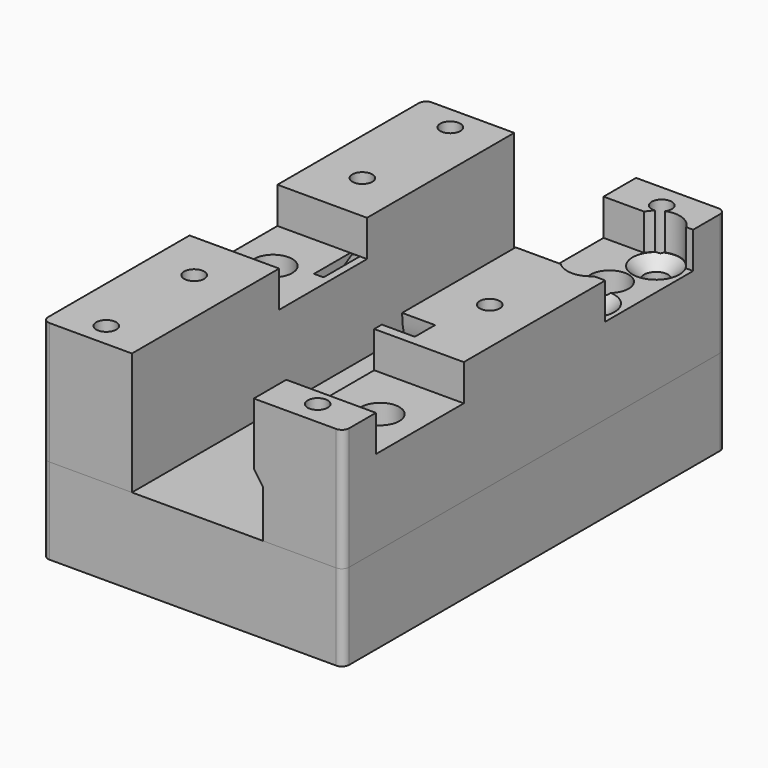
from build123d import *

# Parameters (mm, degrees)
F0_W      = 63
F0_H      = 100
F0_R      = 4
F1_DEPTH  = 25.6
F2_W      = 23
F2_H      = 7.6
F3_DEPTH  = 31.501
F4_W      = 23
F4_H      = 7.6
F5_DEPTH  = 31.501
F6_W      = 25.5
F6_H      = 100
F7_DEPTH  = 25.601
F8_R      = 4
F9_DEPTH  = 17
F10_R     = 2.1
F11_DEPTH = 29
F13_DEPTH = 100.001
F15_DEPTH = 15
F16_DEPTH = 5
F17_R     = 2.5
F18_DEPTH = 15.601
F20_DEPTH = 7.6
F22_R     = 1.5
F23_W     = 2
F23_H     = 20
F24_DEPTH = 18
F26_DEPTH = 6.5
F27_W     = 2
F27_H     = 20
F28_DEPTH = 3
F29_R     = 2.75
F30_DEPTH = 18
F31_R     = 3.4
F32_DEPTH = 43.6010001


# Not quite as in the source:
# - a fillet or chamfer that OpenCascade refuses, or shapes differently, is made with other operations: its cross-section is extruded or revolved along the edge and cut away or added


with BuildPart() as f1:
    # F0 (on Top) → F1 (new body)
    with BuildSketch(Plane.XY):
        Rectangle(F0_W, F0_H)
        with Locations((23.2, -30)):
            Circle(F0_R, mode=Mode.SUBTRACT)
        with Locations((-23.2, 0)):
            Circle(F0_R, mode=Mode.SUBTRACT)
        with Locations((23.2, 30)):
            Circle(F0_R, mode=Mode.SUBTRACT)
    extrude(amount=F1_DEPTH)

    # F2 (on Right) → F3 (cut, through all)
    with BuildSketch(Plane.YZ):
        with Locations((0, 21.8)):
            Rectangle(F2_W, F2_H)
    extrude(amount=-F3_DEPTH, mode=Mode.SUBTRACT)

    # F4 (on Right) → F5 (cut, through all)
    with BuildSketch(Plane.YZ):
        with Locations((-30, 21.8)):
            Rectangle(F4_W, F4_H)
        with Locations((30, 21.8)):
            Rectangle(F4_W, F4_H)
    extrude(amount=F5_DEPTH, mode=Mode.SUBTRACT)

    # F6 (on face) → F7 (cut, through all)
    with BuildSketch(Plane(origin=(0, 0, 0), x_dir=(1, 0, 0), z_dir=(0, 0, -1))):
        Rectangle(F6_W, F6_H)
    extrude(amount=-F7_DEPTH, mode=Mode.SUBTRACT)

    # F8 (on face) → F9 (cut)
    with BuildSketch(Plane(origin=(-31.5, 0, 0), x_dir=(0, -1, 0), z_dir=(-1, 0, 0))):
        with Locations((-12, 10)):
            Circle(F8_R)
    extrude(amount=-F9_DEPTH, mode=Mode.SUBTRACT)

    # F10 (on face) → F11 (cut)
    with BuildSketch(Plane.XY.offset(25.6)):
        with Locations((22.125, -45)):
            Circle(F10_R)
        with Locations((-22.125, -45)):
            Circle(F10_R)
        with Locations((22.125, 0)):
            Circle(F10_R)
        with Locations((-22.125, -22)):
            Circle(F10_R)
        with Locations((-22.125, 22)):
            Circle(F10_R)
        with Locations((-22.125, 45)):
            Circle(F10_R)
        with Locations((22.125, 45)):
            Circle(F10_R)
    extrude(amount=-F11_DEPTH, mode=Mode.SUBTRACT)

    # F12 (on face) → F13 (cut, through all)
    with BuildSketch(Plane.XZ.offset(50)):
        Polygon((12.75, 12.7134812128), (12.75, 0), (14.65, 0), (14.65, 10), align=None)
    extrude(amount=-F13_DEPTH, mode=Mode.SUBTRACT)

    # F14 (on face) → F15 (cut)
    with BuildSketch(Plane(origin=(14.65, 0, 0), x_dir=(0, -1, 0), z_dir=(-1, 0, 0))):
        Polygon((-43.1, 0), (-7.1, 0), (-7.1, 2), (-7.1, 7.3), (-7.1, 10), (-43.1, 10), align=None)
    extrude(amount=-F15_DEPTH, mode=Mode.SUBTRACT)

    # F14 (on face) → F16 (cut, symmetric)
    with BuildSketch(Plane(origin=(14.65, 0, 0), x_dir=(0, -1, 0), z_dir=(-1, 0, 0))):
        Polygon((-43.1, 0), (-7.1, 0), (-7.1, 2), (-7.1, 7.3), (-7.1, 10), (-43.1, 10), align=None)
        with BuildLine():
            Line((-7.1, 7.3), (-7.1, 2))
            ThreePointArc((-7.1, 2), (9.587720036, 8.912279964), (16.5, 25.6))
            Line((16.5, 25.6), (11.2, 25.6))
            ThreePointArc((11.2, 25.6), (5.8400540957, 12.6599459043), (-7.1, 7.3))
        make_face()
    extrude(amount=F16_DEPTH, both=True, mode=Mode.SUBTRACT)

    # F17 (on face) → F18 (cut, through all)
    with BuildSketch(Plane(origin=(0, 0, 10), x_dir=(1, 0, 0), z_dir=(0, 0, -1))):
        with Locations((25.65, -39.1)):
            Circle(F17_R)
        with Locations((25.65, -22.1)):
            Circle(F17_R)
    extrude(amount=-F18_DEPTH, mode=Mode.SUBTRACT)

    # F19 (on face) → F20 (cut, through all)
    with BuildSketch(Plane.XY.offset(18)):
        with BuildLine():
            ThreePointArc((24.95, 41.5), (25.65, 41.6), (26.35, 41.5))
            Line((26.35, 41.5), (30.0363424399, 41.5))
            ThreePointArc((30.0363424399, 41.5), (25.65, 44.1), (21.2636575601, 41.5))
            Line((21.2636575601, 41.5), (24.95, 41.5))
        make_face()
        with BuildLine():
            ThreePointArc((22.1801296854, 18.5), (25.65, 17.1), (29.1198703146, 18.5))
            Line((29.1198703146, 18.5), (22.1801296854, 18.5))
        make_face()
    extrude(amount=F20_DEPTH, mode=Mode.SUBTRACT)

    # F21: chamfer of 2.4 on 2 edges, made by hand

    # F21_s1 → F21_t2 (revolve, cut)
    with BuildSketch(Plane.XZ.offset(-22.1)):
        Polygon((28.15, 15.6), (30.55, 18), (28.15, 18), align=None)
    revolve(axis=Axis((25.65, 22.1, 18), (0, 0, -1)), mode=Mode.SUBTRACT)

    # F21_s3 → F21_t4 (revolve, cut)
    with BuildSketch(Plane.XZ.offset(-39.1)):
        Polygon((28.15, 15.6), (30.55, 18), (28.15, 18), align=None)
    revolve(axis=Axis((25.65, 39.1, 18), (0, 0, -1)), mode=Mode.SUBTRACT)

    # F22
    f22_edges = [f1.edges().sort_by_distance(p)[0] for p in [
        (-31.5, 50, 12.8),
        (31.5, 50, 12.8),
        (31.5, -50, 12.8),
        (-31.5, -50, 12.8),
    ]]
    fillet(f22_edges, radius=F22_R)

    # F23 (on face) → F24 (cut, through all)
    with BuildSketch(Plane(origin=(0, 0, 0), x_dir=(1, 0, 0), z_dir=(0, 0, -1))):
        with Locations((-15.25, -12)):
            Rectangle(F23_W, F23_H)
    extrude(amount=-F24_DEPTH, mode=Mode.SUBTRACT)

    # F25 (on face) → F26 (cut)
    with BuildSketch(Plane.YZ.offset(-16.25)):
        Polygon((5.45, 6.2183557368), (5.45, 0), (18.55, 0), (18.55, 13.7816442632), (12, 17.5632885264), (5.45, 13.7816442632), align=None)
    extrude(amount=-F26_DEPTH, mode=Mode.SUBTRACT)

    # F27 (on face) → F28 (join)
    with BuildSketch(Plane(origin=(0, 0, 0), x_dir=(1, 0, 0), z_dir=(0, 0, -1))):
        with Locations((-15.25, -12)):
            Rectangle(F27_W, F27_H)
    extrude(amount=-F28_DEPTH)


with BuildPart() as f30:
    # F29 (on face) → F30 (new body)
    with BuildSketch(Plane(origin=(0, 0, 0), x_dir=(1, 0, 0), z_dir=(0, 0, -1))):
        with BuildLine():
            ThreePointArc((30, -50), (31.0606601718, -49.5606601718), (31.5, -48.5))
            Line((31.5, -48.5), (31.5, 48.5))
            ThreePointArc((31.5, 48.5), (31.0606601718, 49.5606601718), (30, 50))
            Line((30, 50), (14.65, 50))
            Line((14.65, 50), (-12.75, 50))
            Line((-12.75, 50), (-30, 50))
            ThreePointArc((-30, 50), (-31.0606601718, 49.5606601718), (-31.5, 48.5))
            Line((-31.5, 48.5), (-31.5, -48.5))
            ThreePointArc((-31.5, -48.5), (-31.0606601718, -49.5606601718), (-30, -50))
            Line((-30, -50), (-12.75, -50))
            Line((-12.75, -50), (14.65, -50))
            Line((14.65, -50), (30, -50))
        make_face()
        with Locations((-22.125, -45)):
            Circle(F29_R, mode=Mode.SUBTRACT)
        with Locations((-22.125, -22)):
            Circle(F29_R, mode=Mode.SUBTRACT)
        with Locations((22.125, -45)):
            Circle(F29_R, mode=Mode.SUBTRACT)
        with Locations((-22.125, 22)):
            Circle(F29_R, mode=Mode.SUBTRACT)
        with Locations((-22.125, 45)):
            Circle(F29_R, mode=Mode.SUBTRACT)
        with Locations((22.125, 0)):
            Circle(F29_R, mode=Mode.SUBTRACT)
        with Locations((22.125, 45)):
            Circle(F29_R, mode=Mode.SUBTRACT)
    extrude(amount=F30_DEPTH)

    # F31 (on face) → F32 (cut, through all)
    with BuildSketch(Plane(origin=(0, 0, -18), x_dir=(1, 0, 0), z_dir=(0, 0, -1))):
        with Locations((-20, 35)):
            Circle(F31_R)
        with Locations((20, 35)):
            Circle(F31_R)
        with Locations((20, -35)):
            Circle(F31_R)
        with Locations((-20, -35)):
            Circle(F31_R)
    extrude(amount=-F32_DEPTH, mode=Mode.SUBTRACT)


solid = Compound([f1.part, f30.part])
